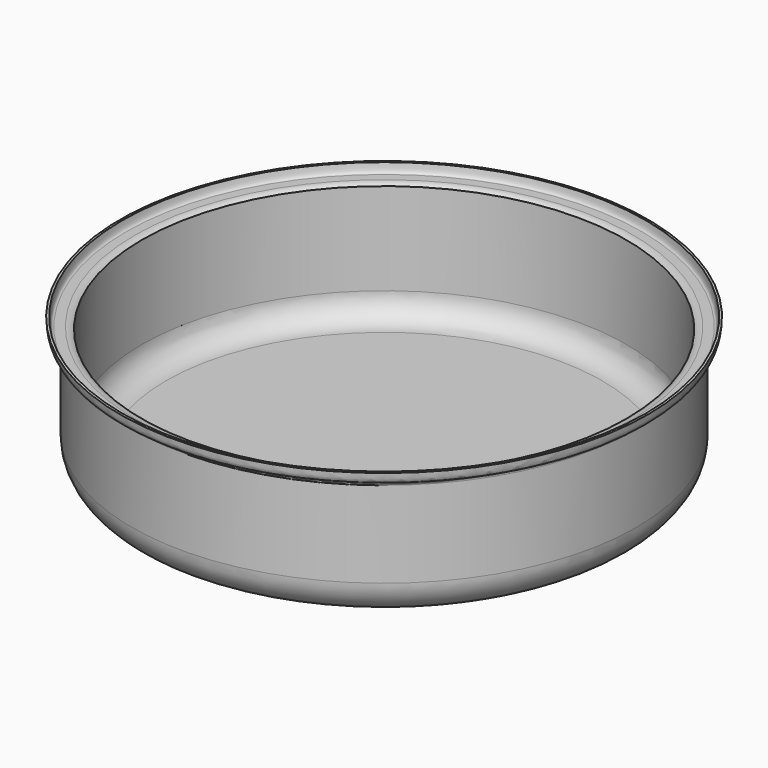
from build123d import *


# Not quite as in the source:
# - ends of sketch curves that miss each other by under 0.0002 mm in the source are joined
# - the dataset's text gives a spline's control points without its knots; the knots are read off the source's solid


with BuildPart() as f1:
    # F0 (on Front) → F1 (revolve)
    with BuildSketch(Plane.XZ):
        with BuildLine():
            ThreePointArc((95, 0), (105.6066017178, 4.3933982822), (110, 15))
            Line((110, 15), (110, 52.530664077))
            ThreePointArc((110, 52.530664077), (110.6656938493, 54.229287327), (112.3082567563, 55.0233001372))
            add(Edge.make_bspline(
                [(112.3082567563, 55.0233001372), (112.3371382541, 55.0255218154), (112.3662455353, 55.0279709343), (112.3956622966, 55.030664077)],
                knots=[0.3810790212, 0.3810790212, 0.3810790212, 0.3810790212, 0.3991629595, 0.3991629595, 0.3991629595, 0.3991629595], degree=3))
            add(Edge.make_bspline(
                [(112.3956622966, 55.030664077), (113.3730312437, 55.1201434726), (114.6920333455, 55.4789992419), (114.9571856025, 59.8162261419)],
                knots=[0.3991629595, 0.3991629595, 0.3991629595, 0.3991629595, 1, 1, 1, 1], degree=3))
            ThreePointArc((114.9571856025, 59.8162261419), (114.4670860694, 59.9975450862), (113.9589484435, 59.8756013901))
            add(Edge.make_bspline(
                [(112.3044930104, 56.0264915082), (112.3140793136, 56.0273704068), (112.3650984167, 56.0322078345), (112.4927350046, 56.0466584989), (112.6564819563, 56.0784065116), (112.8095723323, 56.1345234503), (112.9464281063, 56.217405399), (113.1051907024, 56.367326932), (113.2969685197, 56.6463774626), (113.5030707113, 57.1049132693), (113.7625500872, 57.9971767083), (113.9062854104, 59.0152971487), (113.9589484435, 59.8756013901)],
                knots=[0.3990705563, 0.3990705563, 0.3990705563, 0.3990705563, 0.40625, 0.4375, 0.5, 0.5625, 0.625, 0.6875, 0.75, 0.8125, 0.875, 0.9999203957, 0.9999203957, 0.9999203957, 0.9999203957], degree=3))
            Line((112.3044930104, 56.0264915082), (108.406190974, 56.0264994193))
            ThreePointArc((108.406190974, 56.0264994193), (106.8803038189, 55.787976962), (105.5000000054, 55.0951667753))
            Line((105.5000000054, 55.0951667753), (105.5, 15))
            ThreePointArc((105.5, 15), (102.4246212025, 7.5753787975), (95, 4.5))
            Line((95, 4.5), (92.4233198166, 4.5))
            Line((92.4233198166, 4.5), (0, 4.5))
            Line((0, 4.5), (0, 0))
            Line((0, 0), (92.4233198166, 0))
            Line((92.4233198166, 0), (95, 0))
        make_face()
        with BuildLine():
            add(Edge.make_bspline(
                [(112.3082567563, 55.0233001372), (112.3371382541, 55.0255218154), (112.3662455353, 55.0279709343), (112.3956622966, 55.030664077)],
                knots=[0.3810790212, 0.3810790212, 0.3810790212, 0.3810790212, 0.3991629595, 0.3991629595, 0.3991629595, 0.3991629595], degree=3))
            ThreePointArc((112.3082567563, 55.0233001372), (112.4040577008, 55.0288224137), (112.5, 55.030664077))
            Line((112.5, 55.030664077), (112.3956622966, 55.030664077))
        make_face()
    revolve(axis=Axis((0, 0, 2.25), (0, 0, 1)))


solid = f1.part
